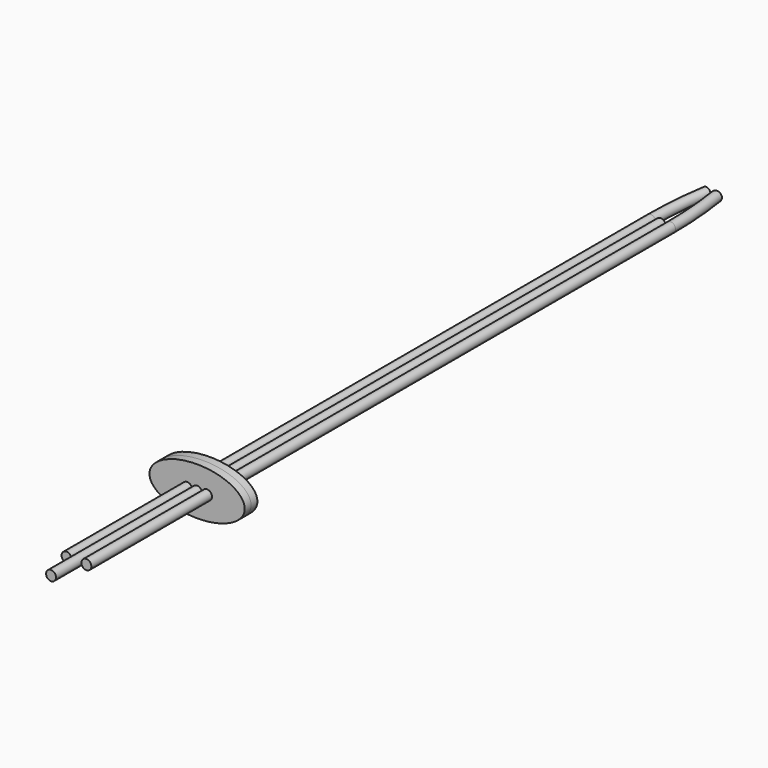
from build123d import *

# Parameters (mm, degrees)
F0_W     = 3.96875
F0_H     = 609.6
F2_R     = 3.96875
F8_DEPTH = 6.35


with BuildPart() as f1:
    # F0 (on Top) → F1 (revolve)
    with BuildSketch(Plane.XY):
        with Locations((-1.984375, 279.4)):
            Rectangle(F0_W, F0_H)
    revolve(axis=Axis((0, 279.4, 0), (0, 1, 0)))


with BuildPart() as f4:
    # F4: sweep along a path in F3
    with BuildLine(Plane.XY) as f4_path:
        Line((7.9375, 0), (7.9375, 584.2))
        ThreePointArc((7.9375, 584.2), (6.9438031447, 609.6773967301), (3.96875, 635))
    # F2 (on Front) → F4 (sweep)
    with BuildSketch(Plane.XZ):
        with Locations((7.9375, 0)):
            Circle(F2_R)
    sweep(path=f4_path.line)


with BuildPart() as f5_1:
    # F5: instance of F4
    add(f4.part.mirror(Plane.YZ))


with BuildPart() as f8:
    # F7 (on offset) → F8 (new body, symmetric)
    with BuildSketch(Plane.XZ.offset(-127)):
        with BuildLine():
            add(Edge.make_bspline(
                [(-38.1, 0), (-38.1, -32.9955678842), (19.05, -16.4977839421), (76.2, 0), (19.05, 16.4977839421), (-38.1, 32.9955678842), (-38.1, 0)],
                knots=[0, 0, 0, 2.0943951024, 2.0943951024, 4.1887902048, 4.1887902048, 6.2831853072, 6.2831853072, 6.2831853072], degree=2, weights=[1, 0.5, 1, 0.5, 1, 0.5, 1]))
        make_face()
    extrude(amount=F8_DEPTH, both=True)


solid = Compound([f1.part, f4.part, f5_1.part, f8.part])
